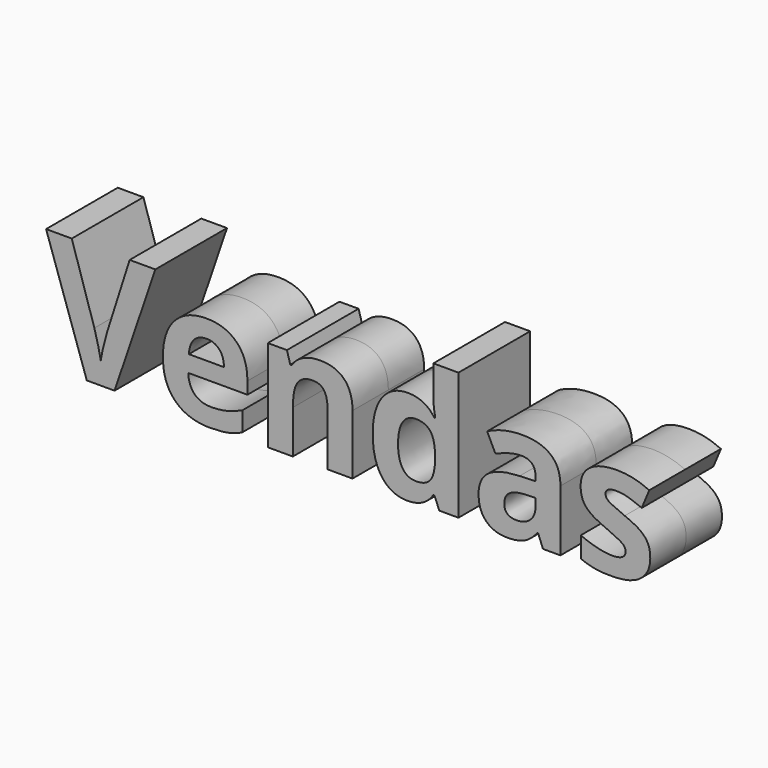
from build123d import *

# Parameters (mm, degrees)
F0_TEXT_SIZE = 112.6040187147
F1_DEPTH     = 30


# Not quite as in the source:
# - Text() gives the source's letters only with a copy of the font that has no kerning and outlines rounded to 1/6400 em; it was checked with that copy


with BuildPart() as f1:
    # F0 (on Front) → F1 (new body, symmetric)
    with BuildSketch(Plane.XZ):
        with Locations((-192.6628649235, 49.2507517338)):
            Text('Vendas', F0_TEXT_SIZE, font='Open Sans', font_style=FontStyle.BOLD, text_align=(TextAlign.LEFT, TextAlign.BOTTOM))
    extrude(amount=F1_DEPTH, both=True)


solid = f1.part
